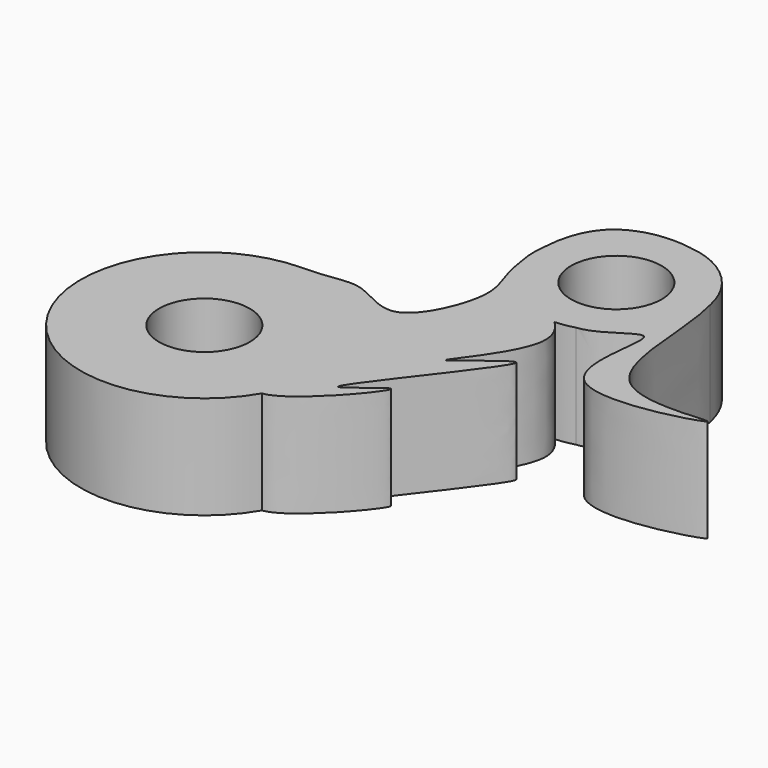
from build123d import *

# Parameters (mm, degrees)
F0_R     = 11
F1_DEPTH = 25


with BuildPart() as f1:
    # F0 (on Top) → F1 (new body)
    with BuildSketch(Plane.XY):
        with BuildLine():
            ThreePointArc((25.9807621135, -15), (28.9777747887, -7.7645713531), (30, 0))
            ThreePointArc((30, 0), (21.2132034356, 21.2132034356), (0, 30))
            ThreePointArc((0, 30), (-25.9807621135, -15), (25.9807621135, -15))
        make_face()
        Circle(F0_R, mode=Mode.SUBTRACT)
        with BuildLine():
            ThreePointArc((0, 30), (21.2132034356, 21.2132034356), (30, 0))
            ThreePointArc((30, 0), (28.9777747887, -7.7645713531), (25.9807621135, -15))
            add(Edge.make_bspline(
                [(50.9773673549, 42.4738754325), (52.4742941954, 41.0051800936), (58.554492977, 33.0019629667), (34.5260407554, 7.6375536887), (70.0809747651, 39.3206227472), (22.9551822625, -16.5311362176), (53.7655390929, 11.9282676195), (32.1412701916, -14.4538743225), (25.9807621135, -15)],
                knots=[0.6922231868, 0.6922231868, 0.6922231868, 0.6922231868, 0.7157925335, 0.7737682263, 0.8203899266, 0.8961903845, 0.9367415839, 1, 1, 1, 1], degree=3))
            ThreePointArc((50.9773673549, 42.4738754325), (37.8467917132, 46.5660406635), (30.4634024291, 58.1696347463))
            add(Edge.make_bspline(
                [(0, 30), (6.7949108517, 30), (12.5283692919, 33.1630296463), (26.5238714057, 21.4790334853), (36.105499568, 44.1712014963), (31.8641340097, 50.1270487683), (30.6380280938, 56.8138647828), (30.4634024291, 58.1696347463)],
                knots=[0, 0, 0, 0, 0.0469677112, 0.091224286, 0.1450750331, 0.189433937, 0.1998528554, 0.1998528554, 0.1998528554, 0.1998528554], degree=3))
        make_face()
        with BuildLine():
            ThreePointArc((30.1803789415, 65.1300212332), (30.0165135371, 61.6374107331), (30.4634024291, 58.1696347463))
            add(Edge.make_bspline(
                [(30.4634024291, 58.1696347463), (30.1836003061, 60.3419804604), (30.0542031477, 62.729768304), (30.1803789415, 65.1300212332)],
                knots=[0.1998528554, 0.1998528554, 0.1998528554, 0.1998528554, 0.2165470538, 0.2165470538, 0.2165470538, 0.2165470538], degree=3))
        make_face()
        with BuildLine():
            add(Edge.make_bspline(
                [(30.4634024291, 58.1696347463), (30.1836003061, 60.3419804604), (30.0542031477, 62.729768304), (30.1803789415, 65.1300212332)],
                knots=[0.1998528554, 0.1998528554, 0.1998528554, 0.1998528554, 0.2165470538, 0.2165470538, 0.2165470538, 0.2165470538], degree=3))
            ThreePointArc((30.4634024291, 58.1696347463), (37.8467917132, 46.5660406635), (50.9773673549, 42.4738754325))
            add(Edge.make_bspline(
                [(55.5760581511, 43.2430131361), (52.0237925534, 42.9082584623), (47.1556867914, 45.3347414454), (49.8993908039, 43.5315217336), (50.9773673549, 42.4738754325)],
                knots=[0.6428347565, 0.6428347565, 0.6428347565, 0.6428347565, 0.6752502778, 0.6922231868, 0.6922231868, 0.6922231868, 0.6922231868], degree=3))
            ThreePointArc((55.5760581511, 43.2430131361), (65.9925164221, 50.4400083567), (70, 62.449979984))
            ThreePointArc((70, 62.449979984), (69.9050330856, 64.3966843425), (69.621034214, 66.3249014505))
            add(Edge.make_bspline(
                [(51.8904656753, 82.3604330057), (57.6411242993, 81.416538227), (65.6845439503, 77.2722836245), (68.9133846164, 69.0394692758), (69.621034214, 66.3249014505)],
                knots=[0.2897570872, 0.2897570872, 0.2897570872, 0.2897570872, 0.324618748, 0.3398287333, 0.3398287333, 0.3398287333, 0.3398287333], degree=3))
            ThreePointArc((51.8904656753, 82.3604330057), (37.5667612566, 78.1156933207), (30.1803789415, 65.1300212332))
        make_face()
        with Locations((50, 62.449979984)):
            Circle(F0_R, mode=Mode.SUBTRACT)
        with BuildLine():
            add(Edge.make_bspline(
                [(55.5760581511, 43.2430131361), (52.0237925534, 42.9082584623), (47.1556867914, 45.3347414454), (49.8993908039, 43.5315217336), (50.9773673549, 42.4738754325)],
                knots=[0.6428347565, 0.6428347565, 0.6428347565, 0.6428347565, 0.6752502778, 0.6922231868, 0.6922231868, 0.6922231868, 0.6922231868], degree=3))
            ThreePointArc((50.9773673549, 42.4738754325), (53.2992028837, 42.7239753117), (55.5760581511, 43.2430131361))
        make_face()
        with BuildLine():
            add(Edge.make_bspline(
                [(30.1803789415, 65.1300212332), (30.4588737331, 70.4278515011), (33.485979065, 81.0744733385), (45.8922083611, 83.3449678443), (51.8904656753, 82.3604330057)],
                knots=[0.2165470538, 0.2165470538, 0.2165470538, 0.2165470538, 0.2533944328, 0.2897570872, 0.2897570872, 0.2897570872, 0.2897570872], degree=3))
            ThreePointArc((30.1803789415, 65.1300212332), (37.5667612566, 78.1156933207), (51.8904656753, 82.3604330057))
        make_face()
        with BuildLine():
            ThreePointArc((70, 62.449979984), (65.9925164221, 50.4400083567), (55.5760581511, 43.2430131361))
            add(Edge.make_bspline(
                [(69.621034214, 66.3249014505), (72.8567075075, 53.9127491013), (68.315749222, 22.9443300379), (116.3570863947, 33.0885115074), (58.8949558462, 15.8977059257), (73.4513604829, 57.0490426254), (61.253618647, 44.0540121965), (55.924524831, 43.275851573), (55.5760581511, 43.2430131361)],
                knots=[0.3398287333, 0.3398287333, 0.3398287333, 0.3398287333, 0.4093752199, 0.4674153296, 0.5357408659, 0.5946800577, 0.6396548903, 0.6428347565, 0.6428347565, 0.6428347565, 0.6428347565], degree=3))
            ThreePointArc((69.621034214, 66.3249014505), (69.9050330856, 64.3966843425), (70, 62.449979984))
        make_face()
        with BuildLine():
            ThreePointArc((69.621034214, 66.3249014505), (63.4153168035, 77.2833637875), (51.8904656753, 82.3604330057))
            add(Edge.make_bspline(
                [(51.8904656753, 82.3604330057), (57.6411242993, 81.416538227), (65.6845439503, 77.2722836245), (68.9133846164, 69.0394692758), (69.621034214, 66.3249014505)],
                knots=[0.2897570872, 0.2897570872, 0.2897570872, 0.2897570872, 0.324618748, 0.3398287333, 0.3398287333, 0.3398287333, 0.3398287333], degree=3))
        make_face()
    extrude(amount=F1_DEPTH)


solid = f1.part
